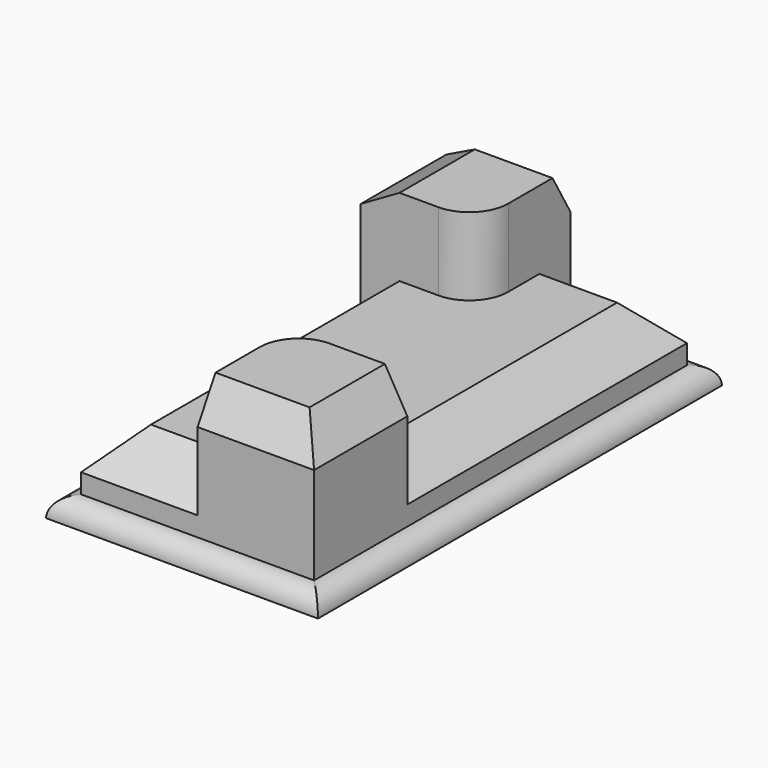
from build123d import *

# Parameters (mm, degrees)
F0_W        = 88.9
F0_H        = 165.1
F1_DEPTH    = 6.35
F2_DEPTH    = 25.4
F3_DEPTH    = 50.8
F4_R        = 6.34999
F5_SIZE2    = 12.7
F5_SIZE     = 12.7
F6_C1_SIZE2 = 12.7
F6_C1_SIZE  = 7.3323484187
F6_C2_SIZE2 = 7.3323484187
F6_C2_SIZE  = 12.7
F6_C3_SIZE2 = 7.3323484187
F6_C3_SIZE  = 12.7
F6_C4_SIZE2 = 7.3323484187
F6_C4_SIZE  = 12.7


# Not quite as in the source:
# - a fillet or chamfer is up to 0.001 mm smaller than in the source, because OpenCascade refuses the exact size


with BuildPart() as f1:
    # F0 (on Top) → F1 (new body)
    with BuildSketch(Plane.XY):
        with Locations((59.7539862376, 23.8323401288)):
            Rectangle(F0_W, F0_H)
        Polygon((21.6539862376, 61.9323401288), (21.6539862376, 100.0323401288), (59.7539862376, 100.0323401288), (97.8539862376, 100.0323401288), (97.8539862376, -14.2676598712), (97.8539862376, -52.3676598712), (59.7539862376, -52.3676598712), (21.6539862376, -52.3676598712), align=None, mode=Mode.SUBTRACT)
    extrude(amount=F1_DEPTH)

    # F0 (on Top) → F2 (join)
    with BuildSketch(Plane.XY):
        with BuildLine():
            Line((97.8539862376, 100.0323401288), (59.7539862376, 100.0323401288))
            Line((59.7539862376, 100.0323401288), (59.7539862376, 74.6323401288))
            ThreePointArc((59.7539862376, 74.6323401288), (56.0342423587, 65.6520840077), (47.0539862376, 61.9323401288))
            Line((47.0539862376, 61.9323401288), (21.6539862376, 61.9323401288))
            Line((21.6539862376, 61.9323401288), (21.6539862376, -52.3676598712))
            Line((21.6539862376, -52.3676598712), (59.7539862376, -52.3676598712))
            Line((59.7539862376, -52.3676598712), (59.7539862376, -26.9676598712))
            ThreePointArc((59.7539862376, -26.9676598712), (63.4737301166, -17.9874037501), (72.4539862376, -14.2676598712))
            Line((72.4539862376, -14.2676598712), (97.8539862376, -14.2676598712))
            Line((97.8539862376, -14.2676598712), (97.8539862376, 100.0323401288))
        make_face()
    extrude(amount=F2_DEPTH)

    # F0 (on Top) → F3 (join)
    with BuildSketch(Plane.XY):
        with BuildLine():
            Line((59.7539862376, 100.0323401288), (21.6539862376, 100.0323401288))
            Line((21.6539862376, 100.0323401288), (21.6539862376, 61.9323401288))
            Line((21.6539862376, 61.9323401288), (47.0539862376, 61.9323401288))
            ThreePointArc((47.0539862376, 61.9323401288), (56.0342423587, 65.6520840077), (59.7539862376, 74.6323401288))
            Line((59.7539862376, 74.6323401288), (59.7539862376, 100.0323401288))
        make_face()
        with BuildLine():
            Line((97.8539862376, -52.3676598712), (97.8539862376, -14.2676598712))
            Line((97.8539862376, -14.2676598712), (72.4539862376, -14.2676598712))
            ThreePointArc((72.4539862376, -14.2676598712), (63.4737301166, -17.9874037501), (59.7539862376, -26.9676598712))
            Line((59.7539862376, -26.9676598712), (59.7539862376, -52.3676598712))
            Line((59.7539862376, -52.3676598712), (97.8539862376, -52.3676598712))
        make_face()
    extrude(amount=F3_DEPTH)

    # F4 (radius 6.35 in the source; OpenCascade refuses exactly that, so slightly less here)
    f4_edges = [f1.edges().sort_by_distance(p)[0] for p in [
        (15.303986, 23.83234, 6.35),
        (59.753986, 106.38234, 6.35),
        (59.753986, -58.71766, 6.35),
        (104.203986, 23.83234, 6.35),
    ]]
    fillet(f4_edges, radius=F4_R)

    # F5
    f5_edges = [f1.edges().sort_by_distance(p)[0] for p in [
        (21.653986, 4.78234, 25.4),
        (40.703986, -52.36766, 25.4),
        (97.853986, 42.88234, 25.4),
        (78.803986, 100.03234, 25.4),
    ]]
    chamfer(f5_edges, length=F5_SIZE, length2=F5_SIZE2)

    # F6: chamfer of 12.7 x 7.3323484187 on 4 edges, made by hand

    # F6_c1
    f6_c1_edges = [f1.edges().sort_by_distance(p)[0] for p in [
        (21.6539862376, 80.9823401288, 50.8),
    ]]
    f6_c1_side = f1.faces().sort_by_distance((21.6539862376, 80.9823401288, 50.6533530316))[0]
    chamfer(f6_c1_edges, length=F6_C1_SIZE, length2=F6_C1_SIZE2, reference=f6_c1_side)

    # F6_c2
    f6_c2_edges = [f1.edges().sort_by_distance(p)[0] for p in [
        (78.8039862376, -52.3676598712, 50.8),
    ]]
    f6_c2_side = f1.faces().sort_by_distance((78.8039862376, -52.3676598712, 50.6533530316))[0]
    chamfer(f6_c2_edges, length=F6_C2_SIZE, length2=F6_C2_SIZE2, reference=f6_c2_side)

    # F6_c3
    f6_c3_edges = [f1.edges().sort_by_distance(p)[0] for p in [
        (47.0539862376, 100.0323401288, 50.8),
    ]]
    f6_c3_side = f1.faces().sort_by_distance((47.0539862376, 100.0323401288, 50.6533530316))[0]
    chamfer(f6_c3_edges, length=F6_C3_SIZE, length2=F6_C3_SIZE2, reference=f6_c3_side)

    # F6_c4
    f6_c4_edges = [f1.edges().sort_by_distance(p)[0] for p in [
        (97.8539862376, -29.6514856618, 50.8),
    ]]
    f6_c4_side = f1.faces().sort_by_distance((97.8539862376, -29.6514856618, 50.6533530316))[0]
    chamfer(f6_c4_edges, length=F6_C4_SIZE, length2=F6_C4_SIZE2, reference=f6_c4_side)


solid = f1.part
